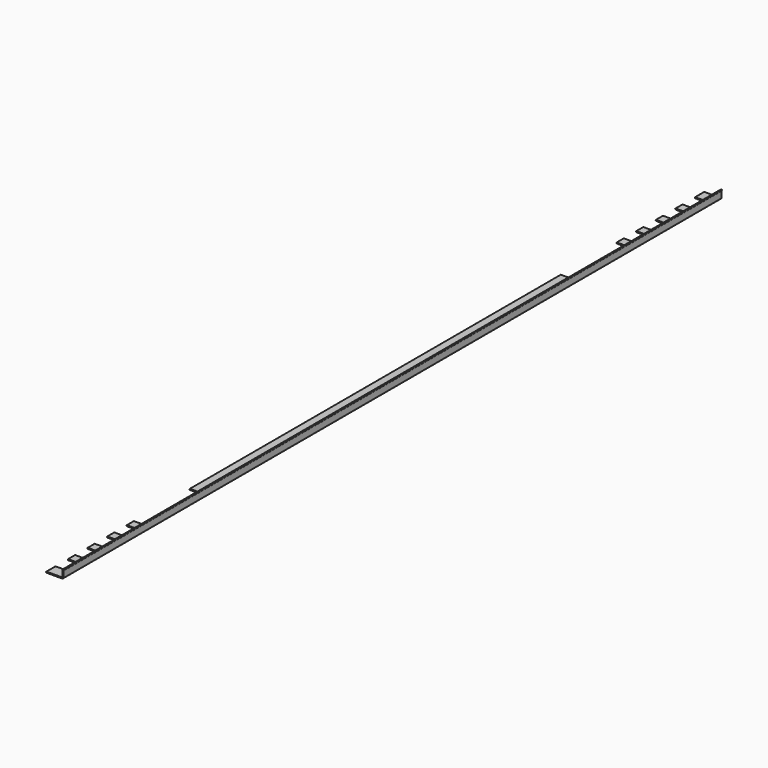
from build123d import *

# Parameters (mm, degrees)
F1_DEPTH = 596.9
F2_R     = 0.76199
F3_W     = 50.8
F3_H     = 101.6
F4_DEPTH = 1.525
F5_W     = 50.8
F5_H     = 22.86
F6_DEPTH = 1.525
F7_R     = 3.175


# Not quite as in the source:
# - a fillet or chamfer is up to 0.001 mm smaller than in the source, because OpenCascade refuses the exact size


with BuildPart() as f1:
    # F0 (on Front) → F1 (new body)
    with BuildSketch(Plane.XZ):
        with BuildLine():
            Line((1.524, 0.762), (1.524, 9.0941772846))
            ThreePointArc((1.524, 9.0941772846), (1.6260886423, 9.4751772846), (1.905, 9.7540886423))
            ThreePointArc((1.905, 9.7540886423), (2.2600354796, 10.6112201124), (1.524, 11.176))
            ThreePointArc((1.524, 11.176), (0.4463692655, 10.7296307345), (0, 9.652))
            Line((0, 9.652), (0, 0.762))
            ThreePointArc((0, 0.762), (-0.2231846327, 0.2231846327), (-0.762, 0))
            Line((-0.762, 0), (-23.876, 0))
            Line((-23.876, 0), (-23.876, -1.524))
            Line((-23.876, -1.524), (-0.762, -1.524))
            ThreePointArc((-0.762, -1.524), (0.8544461018, -0.8544461018), (1.524, 0.762))
        make_face()
    extrude(amount=F1_DEPTH)

    # F2 (radius 0.762 in the source; OpenCascade refuses exactly that, so slightly less here)
    f2_edges = [f1.edges().sort_by_distance(p)[0] for p in [
        (-23.876, -298.45, 0),
        (-23.876, -298.45, -1.524),
    ]]
    fillet(f2_edges, radius=F2_R)

    # F3 (on Top) → F4 (cut, through all)
    with BuildSketch(Plane.XY):
        with Locations((-26.924, -387.35)):
            Rectangle(F3_W, F3_H)
    extrude(amount=-F4_DEPTH, mode=Mode.SUBTRACT)

    # F5 (on Top) → F6 (cut, through all)
    with BuildSketch(Plane.XY):
        with Locations((-26.924, -462.28)):
            Rectangle(F5_W, F5_H)
        with Locations((-26.924, -497.84)):
            Rectangle(F5_W, F5_H)
        with Locations((-26.924, -533.4)):
            Rectangle(F5_W, F5_H)
        with Locations((-26.924, -568.96)):
            Rectangle(F5_W, F5_H)
    extrude(amount=-F6_DEPTH, mode=Mode.SUBTRACT)

    # F7
    f7_edges = [f1.edges().sort_by_distance(p)[0] for p in [
        (-1.524, -336.55, -0.762),
        (-1.524, -438.15, -0.762),
        (-1.524, -450.85, -0.762),
        (-1.524, -473.71, -0.762),
        (-1.524, -509.27, -0.762),
        (-1.524, -544.83, -0.762),
        (-1.524, -580.39, -0.762),
        (-1.524, -486.41, -0.762),
        (-1.524, -521.97, -0.762),
        (-1.524, -557.53, -0.762),
    ]]
    fillet(f7_edges, radius=F7_R)

    # F8: F1 across plane


with BuildPart() as f1_1:
    add(f1.part)
    add(f1.part.mirror(Plane.XZ))


solid = f1_1.part
